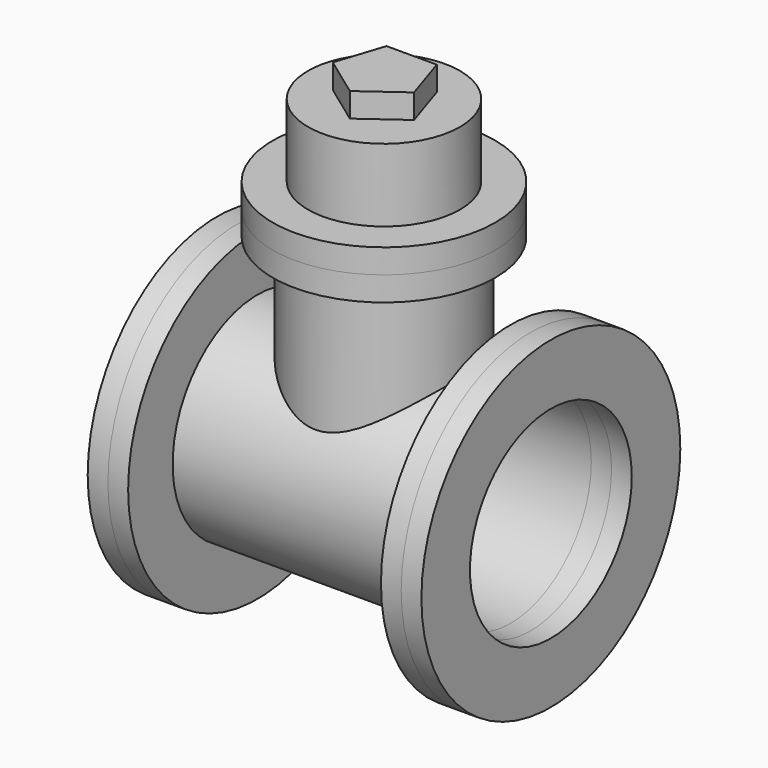
from build123d import *

# Parameters (mm, degrees)
F0_R      = 203.2
F0_R_2    = 127
F1_DEPTH  = 25.4
F3_R      = 203.2
F3_R_2    = 127
F4_DEPTH  = 25.4
F6_DEPTH  = 25.4
F7_DEPTH  = 25.4
F9_R      = 133.35
F9_R_2    = 127
F10_DEPTH = 317.5
F12_R     = 139.7
F13_DEPTH = 30.48
F14_R     = 107.3588969204
F15_REACH = 755.7778161324
F16_DEPTH = 30.48
F17_R     = 95.4249040927
F18_DEPTH = 91.44
F20_DEPTH = 30.48


with BuildPart() as f1:
    # F0 (on Right) → F1 (new body)
    with BuildSketch(Plane.YZ):
        Circle(F0_R)
        Circle(F0_R_2, mode=Mode.SUBTRACT)
    extrude(amount=F1_DEPTH)


with BuildPart() as f4:
    # F3 (on offset) → F4 (new body)
    with BuildSketch(Plane.YZ.offset(-317.5)):
        Circle(F3_R)
        Circle(F3_R_2, mode=Mode.SUBTRACT)
    extrude(amount=-F4_DEPTH)


with BuildPart() as f6:
    # F6 (new): a face of the model
    f6_faces = [f4.part.faces().sort_by_distance(p)[0] for p in [
        (-342.9, -197.4526360825, 0),
    ]]
    extrude(f6_faces, amount=F6_DEPTH)


with BuildPart() as f7:
    # F7 (new): a face of the model
    f7_faces = [f1.part.faces().sort_by_distance(p)[0] for p in [
        (25.4, -197.4526360825, 0),
    ]]
    extrude(f7_faces, amount=F7_DEPTH)


with BuildPart() as f1_1:
    add(f1.part)

    add(f4.part)  # F10 merges F4
    # F9 (on face) → F10 (join, through all)
    with BuildSketch(Plane.YZ.offset(-317.5)):
        Circle(F9_R)
        Circle(F9_R_2, mode=Mode.SUBTRACT)
    extrude(amount=F10_DEPTH)



with BuildPart() as f13:
    # F12 (on offset) → F13 (new body)
    with BuildSketch(Plane.XY.offset(279.4)):
        with Locations((-158.75, 0)):
            Circle(F12_R)
    extrude(amount=-F13_DEPTH)


with BuildPart() as f1_2:
    add(f1_1.part)

    add(f13.part)  # F15 merges F13
    f15_end = f1_2.faces().sort_by_distance((-158.75, -133.35, 0))[0]
    # F14 (on face) → F15 (join, up to a face of the model that its end follows)
    with BuildSketch(Plane(origin=(0, 0, 248.92), x_dir=(1, 0, 0), z_dir=(0, 0, -1))):
        with Locations((-158.75, 0)):
            Circle(F14_R)
    f15_long = extrude(amount=F15_REACH, mode=Mode.PRIVATE)
    add(split(f15_long, bisect_by=f15_end, keep=Keep.ALL, mode=Mode.PRIVATE).solids().sort_by_distance((-158.75, 0, 248.92))[0])


with BuildPart() as f16:
    # F16 (new): a face of the model
    f16_faces = [f1_2.part.faces().sort_by_distance(p)[0] for p in [
        (-158.75, 0, 279.4),
    ]]
    extrude(f16_faces, amount=F16_DEPTH)

    # F17 (on face) → F18 (join)
    with BuildSketch(Plane.XY.offset(309.88)):
        with Locations((-158.75, 0)):
            Circle(F17_R)
    extrude(amount=F18_DEPTH)

    # F19 (on face) → F20 (join)
    with BuildSketch(Plane.XY.offset(401.32)):
        Polygon((-127.2176910353, 43.4004999697), (-190.2823089647, 43.4004999697), (-209.7703476486, -16.5775158597), (-158.75, -53.6459682201), (-107.7296523514, -16.5775158597), align=None)
    extrude(amount=F20_DEPTH)


solid = Compound([f6.part, f7.part, f1_2.part, f16.part])
